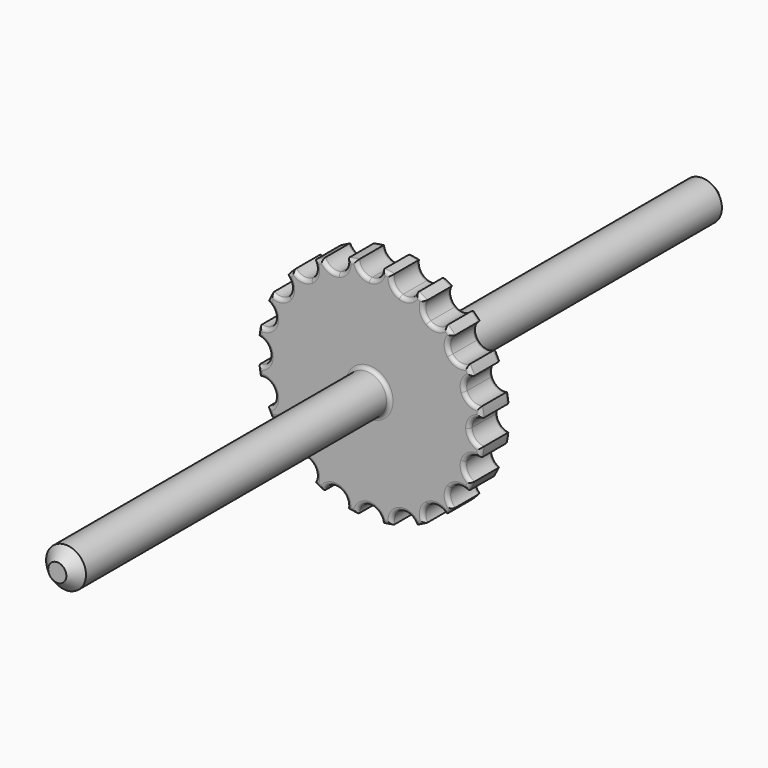
from build123d import *

# Parameters (mm, degrees)
F0_R            = 310
F0_R_2          = 55
F1_DEPTH        = 50
F2_DEPTH        = 1125
F3_SIZE         = 30
F5_DEPTH        = 100
F5_COPIES_COUNT = 20
F6_R            = 10
F7_R            = 10


# Not quite as in the source:
# - a pattern or mirror of a feature is missing from the dataset's text; its kind, count and spacing are read off the source's solid


with BuildPart() as f1:
    # F0 (on Front) → F1 (new body, symmetric)
    with BuildSketch(Plane.XZ):
        Circle(F0_R)
        Circle(F0_R_2, mode=Mode.SUBTRACT)
    extrude(amount=F1_DEPTH, both=True)

    # F0 (on Front) → F2 (join, symmetric)
    with BuildSketch(Plane.XZ):
        Circle(F0_R_2)
    extrude(amount=F2_DEPTH, both=True)

    # F3
    f3_edges = [f1.edges().sort_by_distance(p)[0] for p in [
        (-55, -1125, 0),
        (-55, 1125, 0),
    ]]
    chamfer(f3_edges, length=F3_SIZE)

    # F4 (on face) → F5 (cut)
    with BuildSketch(Plane(origin=(0, 50, 0), x_dir=(-1, 0, 0), z_dir=(0, 1, 0))):
        with BuildLine():
            ThreePointArc((34.9441867678, -308.0241935484), (24.0400370741, -284.5622992887), (-2.618e-07, -275))
            ThreePointArc((-2.618e-07, -275), (-24.0400372643, -284.5622994685), (-34.9441867678, -308.0241935484))
            ThreePointArc((-34.9441867678, -308.0241935484), (0, -310), (34.9441867678, -308.0241935484))
        make_face()
    f5 = extrude(amount=-F5_DEPTH, mode=Mode.SUBTRACT)

    # F5_copies: F5 ×20 about axis
    f5_copies_axis = Axis((0, 0, 0), (0, 1, 0))
    for i in range(1, F5_COPIES_COUNT):
        add(f5.rotate(f5_copies_axis, i * 360 / F5_COPIES_COUNT), mode=Mode.SUBTRACT)

    # F6
    f6_edges = [f1.edges().sort_by_distance(p)[0] for p in [
        (0, 50, -275),
        (-48.494684, 50, -306.183386),
        (-84.979673, 50, -261.540542),
        (-140.737055, 50, -276.212022),
        (-161.640944, 50, -222.479673),
        (-219.203102, 50, -219.203102),
        (-222.479673, 50, -161.640944),
        (-276.212022, 50, -140.737055),
        (-261.540542, 50, -84.979673),
        (-306.183386, 50, -48.494684),
        (-275, 50, 0),
        (-306.183386, 50, 48.494684),
        (-261.540542, 50, 84.979673),
        (-276.212022, 50, 140.737055),
        (-222.479673, 50, 161.640944),
        (-219.203102, 50, 219.203102),
        (-161.640944, 50, 222.479673),
        (-140.737055, 50, 276.212022),
        (-84.979673, 50, 261.540542),
        (-48.494684, 50, 306.183386),
        (0, 50, 275),
        (48.494684, 50, 306.183386),
        (84.979673, 50, 261.540542),
        (140.737055, 50, 276.212022),
        (161.640944, 50, 222.479673),
        (219.203102, 50, 219.203102),
        (222.479673, 50, 161.640944),
        (276.212022, 50, 140.737055),
        (261.540542, 50, 84.979673),
        (306.183386, 50, 48.494684),
        (275, 50, 0),
        (306.183386, 50, -48.494684),
        (261.540542, 50, -84.979673),
        (276.212022, 50, -140.737055),
        (222.479673, 50, -161.640944),
        (219.203102, 50, -219.203102),
        (161.640944, 50, -222.479673),
        (140.737055, 50, -276.212022),
        (84.979673, 50, -261.540542),
        (48.494684, 50, -306.183386),
        (-55, 50, 0),
    ]]
    fillet(f6_edges, radius=F6_R)

    # F7
    f7_edges = [f1.edges().sort_by_distance(p)[0] for p in [
        (-48.494684, -50, -306.183386),
        (-84.979673, -50, -261.540542),
        (-140.737055, -50, -276.212022),
        (-161.640944, -50, -222.479673),
        (-219.203102, -50, -219.203102),
        (-222.479673, -50, -161.640944),
        (-276.212022, -50, -140.737055),
        (-261.540542, -50, -84.979673),
        (-306.183386, -50, -48.494684),
        (-275, -50, 0),
        (-306.183386, -50, 48.494684),
        (-261.540542, -50, 84.979673),
        (-276.212022, -50, 140.737055),
        (-222.479673, -50, 161.640944),
        (-219.203102, -50, 219.203102),
        (-161.640944, -50, 222.479673),
        (-140.737055, -50, 276.212022),
        (-84.979673, -50, 261.540542),
        (-48.494684, -50, 306.183386),
        (0, -50, 275),
        (48.494684, -50, 306.183386),
        (84.979673, -50, 261.540542),
        (140.737055, -50, 276.212022),
        (161.640944, -50, 222.479673),
        (219.203102, -50, 219.203102),
        (222.479673, -50, 161.640944),
        (276.212022, -50, 140.737055),
        (261.540542, -50, 84.979673),
        (306.183386, -50, 48.494684),
        (275, -50, 0),
        (306.183386, -50, -48.494684),
        (261.540542, -50, -84.979673),
        (276.212022, -50, -140.737055),
        (222.479673, -50, -161.640944),
        (219.203102, -50, -219.203102),
        (161.640944, -50, -222.479673),
        (140.737055, -50, -276.212022),
        (84.979673, -50, -261.540542),
        (48.494684, -50, -306.183386),
        (0, -50, -275),
        (-55, -50, 0),
    ]]
    fillet(f7_edges, radius=F7_R)


solid = f1.part
